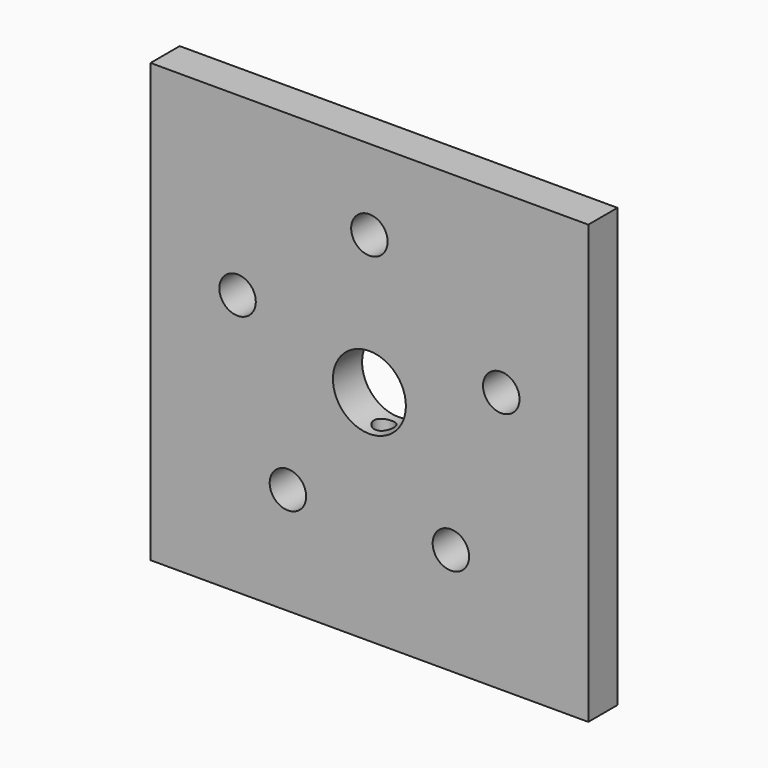
from build123d import *

# Parameters (mm, degrees)
F0_W     = 76.2
F0_H     = 76.2
F0_R     = 3.175
F0_R_2   = 6.35
F1_DEPTH = 6.35
F2_R     = 2.15265
F3_DEPTH = 25.4
F4_R     = 1.7272
F5_REACH = 81.0862593299


with BuildPart() as f1:
    # F0 (on Front) → F1 (new body)
    with BuildSketch(Plane.XZ):
        Rectangle(F0_W, F0_H)
        with Locations((-14.1832581378, -19.5215800743)):
            Circle(F0_R, mode=Mode.SUBTRACT)
        with Locations((14.1832581378, -19.5215800743)):
            Circle(F0_R, mode=Mode.SUBTRACT)
        with Locations((-22.9489937382, 7.4565800743)):
            Circle(F0_R, mode=Mode.SUBTRACT)
        Circle(F0_R_2, mode=Mode.SUBTRACT)
        with Locations((22.9489937382, 7.4565800743)):
            Circle(F0_R, mode=Mode.SUBTRACT)
        with Locations((0, 24.13)):
            Circle(F0_R, mode=Mode.SUBTRACT)
    extrude(amount=F1_DEPTH)

    # F2 (on face) → F3 (cut)
    with BuildSketch(Plane(origin=(0, 0, -38.1), x_dir=(1, 0, 0), z_dir=(0, 0, -1))):
        with Locations((0, 3.175)):
            Circle(F2_R)
    extrude(amount=-F3_DEPTH, mode=Mode.SUBTRACT)

    f5_end = f1.faces().sort_by_distance((-6.35, -3.175, 0))[0]
    # F4 (on face) → F5 (cut, up to a face of the model that its end follows)
    with BuildSketch(Plane(origin=(0, 0, -38.1), x_dir=(1, 0, 0), z_dir=(0, 0, -1))):
        with Locations((0, 3.175)):
            Circle(F4_R)
    f5_long = extrude(amount=-F5_REACH, mode=Mode.PRIVATE)
    add(split(f5_long, bisect_by=f5_end, keep=Keep.ALL, mode=Mode.PRIVATE).solids().sort_by_distance((0, -3.175, -38.1))[0], mode=Mode.SUBTRACT)


solid = f1.part
